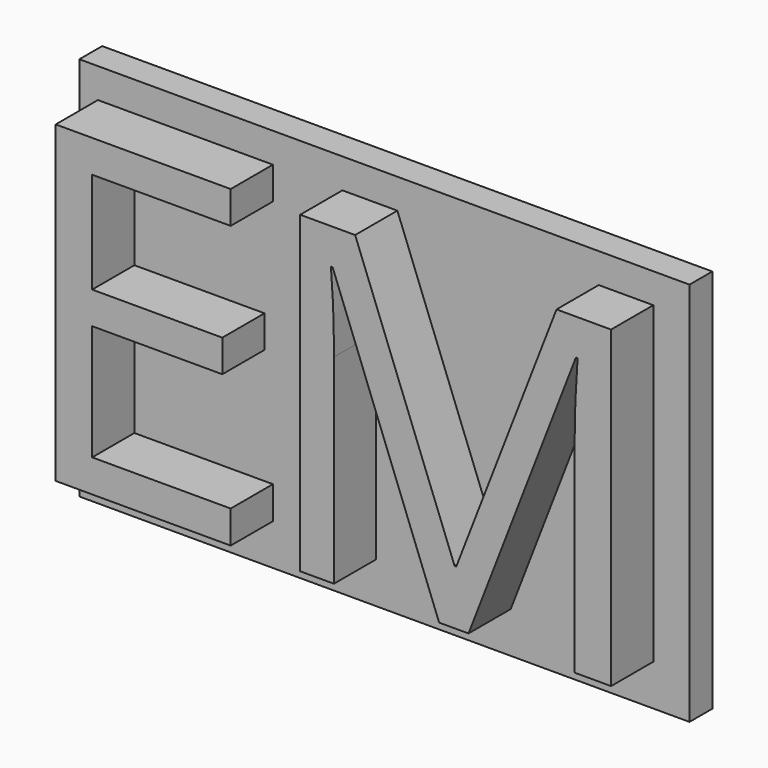
from build123d import *

# Parameters (mm, degrees)
F0_TEXT_SIZE = 105.8333333333
F1_DEPTH     = 12.7
F2_W         = 146.8676663935
F2_H         = 92.6641337574
F3_DEPTH     = 6.858


# Not quite as in the source:
# - Text() gives the source's letters only with a copy of the font that has no kerning and outlines rounded to 1/6400 em; it was checked with that copy


with BuildPart() as f1:
    # F0 (on Front) → F1 (new body)
    with BuildSketch(Plane.XZ):
        with Locations((-51.1840168467, -42.2967627909)):
            Text('EM', F0_TEXT_SIZE, font='Open Sans', text_align=(TextAlign.LEFT, TextAlign.BOTTOM))
    extrude(amount=F1_DEPTH)

    # F2 (on Front) → F3 (join)
    with BuildSketch(Plane.XZ):
        with Locations((28.1689297408, -5.8786924928)):
            Rectangle(F2_W, F2_H)
    extrude(amount=-F3_DEPTH)


solid = f1.part
